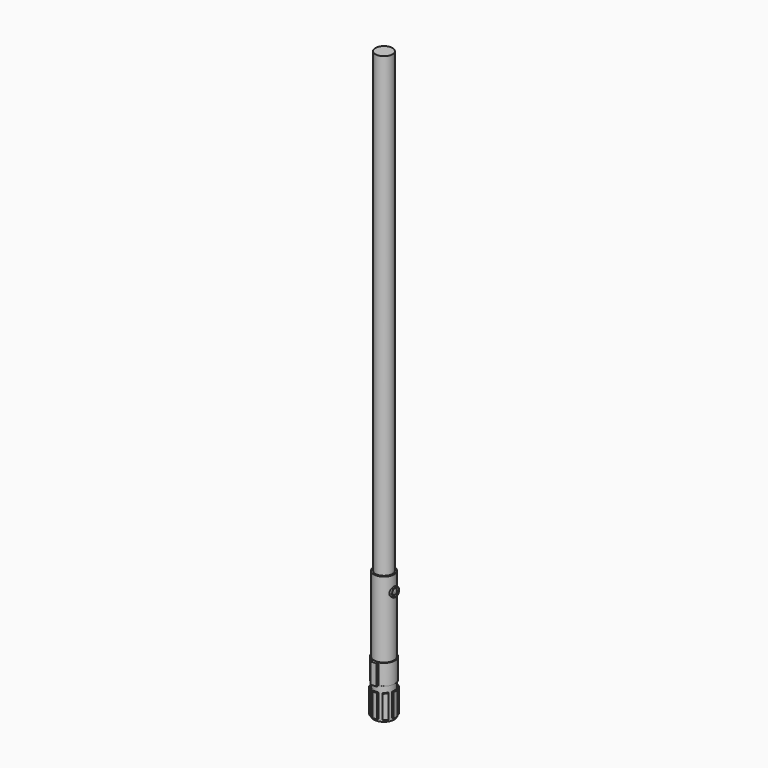
from build123d import *

# Parameters (mm, degrees)
F1_R      = 22.225
F2_DEPTH  = 139.7
F3_W      = 10.16
F3_H      = 50.8
F6_COUNT  = 8
F8_R      = 22.225
F9_DEPTH  = 44.45
F10_R     = 10.16
F10_R_2   = 6.35
F11_REACH = 79.5378195874
F12_SIZE  = 2.54
F13_R     = 0.762
F14_R     = 5.715
F15_REACH = 66.9654610179
F16_R     = 2.54
F17_R     = 18.669
F18_DEPTH = 1000


with BuildPart() as f2:
    # F1 (on Top) → F2 (new body, symmetric)
    with BuildSketch(Plane.XY):
        Circle(F1_R)
    extrude(amount=F2_DEPTH, both=True)


with BuildPart() as f4:
    # F3 (on offset) → F4 (new body, up to the next surface of F2)
    with BuildSketch(Plane.YZ.offset(25.4)):
        with Locations((0, -109.22)):
            Rectangle(F3_W, F3_H)
    extrude(until=Until.NEXT, target=f2.part, dir=(-1, 0, 0))


with BuildPart() as f6_1:
    # F6: instance of F4
    add(f4.part.rotate(Axis((0, 0, 15.8496), (0, 0, -1)), 1 * 360 / F6_COUNT))


with BuildPart() as f6_2:
    # F6: instance of F4
    add(f4.part.rotate(Axis((0, 0, 15.8496), (0, 0, -1)), 2 * 360 / F6_COUNT))


with BuildPart() as f6_3:
    # F6: instance of F4
    add(f4.part.rotate(Axis((0, 0, 15.8496), (0, 0, -1)), 3 * 360 / F6_COUNT))


with BuildPart() as f6_4:
    # F6: instance of F4
    add(f4.part.rotate(Axis((0, 0, 15.8496), (0, 0, -1)), 4 * 360 / F6_COUNT))


with BuildPart() as f6_5:
    # F6: instance of F4
    add(f4.part.rotate(Axis((0, 0, 15.8496), (0, 0, -1)), 5 * 360 / F6_COUNT))


with BuildPart() as f6_6:
    # F6: instance of F4
    add(f4.part.rotate(Axis((0, 0, 15.8496), (0, 0, -1)), 6 * 360 / F6_COUNT))


with BuildPart() as f6_7:
    # F6: instance of F4
    add(f4.part.rotate(Axis((0, 0, 15.8496), (0, 0, -1)), 7 * 360 / F6_COUNT))


with BuildPart() as f9:
    # F8 (on offset) → F9 (new body)
    with BuildSketch(Plane.XY.offset(-25.4)):
        with BuildLine():
            Line((6.35, -28.3594845304), (6.35, -23.2794845304))
            ThreePointArc((6.35, -23.2794845304), (0, 24.13), (-6.35, -23.2794845304))
            Line((-6.35, -23.2794845304), (-6.35, -28.3594845304))
            Line((-6.35, -28.3594845304), (6.35, -28.3594845304))
        make_face()
        Circle(F8_R, mode=Mode.SUBTRACT)
    extrude(amount=-F9_DEPTH)


with BuildPart() as f11:
    f11_end = f2.part.faces().sort_by_distance((-22.225, 0, 0))[0]
    # F10 (on offset) → F11 (new body, up to a face of F2 that its end follows)
    with BuildSketch(Plane.YZ.offset(25.4)):
        with Locations((0, 106.68)):
            Circle(F10_R)
        with Locations((0, 106.68)):
            Circle(F10_R_2, mode=Mode.SUBTRACT)
    f11_long = extrude(amount=-F11_REACH, mode=Mode.PRIVATE)
    add(split(f11_long, bisect_by=f11_end, keep=Keep.ALL, mode=Mode.PRIVATE).solids().sort_by_distance((25.4, -9.8726318041, 106.68))[0])

    # F12
    f12_edges = [f11.edges().sort_by_distance(p)[0] for p in [
        (25.4, -6.35, 106.68),
    ]]
    chamfer(f12_edges, length=F12_SIZE)

    # F13
    f13_edges = [f11.edges().sort_by_distance(p)[0] for p in [
        (24.13, 7.62, 106.68),
        (25.4, -8.89, 106.68),
        (22.86, -6.35, 106.68),
        (25.4, -10.16, 106.68),
    ]]
    fillet(f13_edges, radius=F13_R)


with BuildPart() as f15:
    f15_end = f2.part.faces().sort_by_distance((-22.225, 0, 0))[0]
    # F14 (on offset) → F15 (new body, up to a face of F2 that its end follows)
    with BuildSketch(Plane.YZ.offset(25.4)):
        with Locations((0, 106.68)):
            Circle(F14_R)
    f15_long = extrude(amount=-F15_REACH, mode=Mode.PRIVATE)
    add(split(f15_long, bisect_by=f15_end, keep=Keep.ALL, mode=Mode.PRIVATE).solids().sort_by_distance((25.4, 0, 106.68))[0])

    # F16
    f16_edges = [f15.edges().sort_by_distance(p)[0] for p in [
        (25.4, -5.715, 106.68),
    ]]
    fillet(f16_edges, radius=F16_R)


with BuildPart() as f18:
    # F17 (on face) → F18 (new body)
    with BuildSketch(Plane.XY.offset(139.7)):
        Circle(F17_R)
    extrude(amount=F18_DEPTH)


solid = Compound([f2.part, f4.part, f6_1.part, f6_2.part, f6_3.part, f6_4.part, f6_5.part, f6_6.part, f6_7.part, f9.part, f11.part, f15.part, f18.part])
